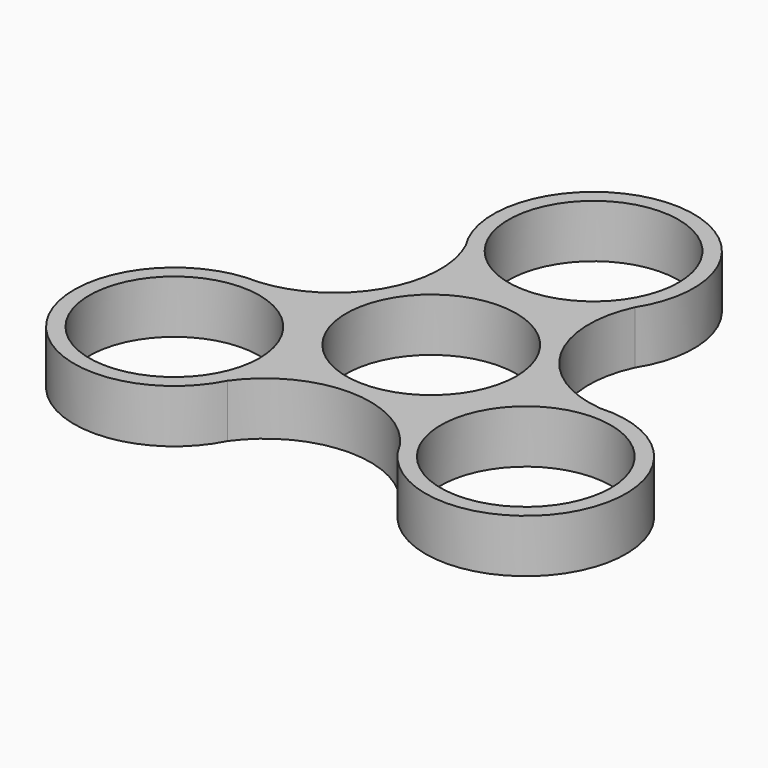
from build123d import *

# Parameters (mm, degrees)
F0_R     = 11.2
F1_DEPTH = 7
F2_R     = 1.5
F3_DEPTH = 7


# Not quite as in the source:
# - a feature names something its author has since deleted; it is built from what else it names


with BuildPart() as f1:
    # F0 (on Top) → F1 (new body)
    with BuildSketch(Plane.XY):
        with BuildLine():
            ThreePointArc((22.3972222345, -0.1780444605), (11.6219084102, 6.8053952105), (11.1419447663, 19.6368196267))
            ThreePointArc((11.1419447663, 19.6368196267), (-0.0899760733, 39.914441113), (-11.0444200915, 19.4855856595))
            ThreePointArc((-11.0444200915, 19.4855856595), (-11.7045993402, 6.6621703185), (-22.5769570295, -0.1692025982))
            ThreePointArc((-22.5769570295, -0.1692025982), (-34.5219319451, -20.0351421217), (-11.352802143, -19.3075411991))
            ThreePointArc((-11.352802143, -19.3075411991), (0.08269093, -13.467565529), (11.4350122631, -19.4676170286))
            ThreePointArc((11.4350122631, -19.4676170286), (34.6119080183, -19.8792989913), (22.3972222345, -0.1780444605))
        make_face()
        with Locations((-23.1356502259, -13.3573738858)):
            Circle(F0_R, mode=Mode.SUBTRACT)
        with Locations((23.1356502259, -13.3573738858)):
            Circle(F0_R, mode=Mode.SUBTRACT)
        Circle(F0_R, mode=Mode.SUBTRACT)
        with Locations((0, 26.7147477716)):
            Circle(F0_R, mode=Mode.SUBTRACT)
    extrude(amount=F1_DEPTH)

    # F2 (call 1 of 2: OpenCascade refuses the feature's edges together)
    f2_edges = [f1.edges().sort_by_distance(p)[0] for p in [
        (-34.521932, -20.035142, 7),
        (-11.704599, 6.66217, 7),
        (34.611908, -19.879299, 7),
        (-0.089976, 39.914441, 7),
        (0.082691, -13.467566, 7),
        (11.621908, 6.805395, 7),
    ]]
    fillet(f2_edges, radius=F2_R)

    # F2#2 (call 2 of 2)
    f2_2_edges = [f1.edges().sort_by_distance(p)[0] for p in [
        (34.611908, -19.879299, 0),
        (0.082691, -13.467566, 0),
        (-34.521932, -20.035142, 0),
        (-0.089976, 39.914441, 0),
        (11.621908, 6.805395, 0),
        (-11.704599, 6.66217, 0),
    ]]
    fillet(f2_2_edges, radius=F2_R)

    # F0 (on Top) → F3 (join)
    with BuildSketch(Plane.XY):
        with BuildLine():
            ThreePointArc((22.3972222345, -0.1780444605), (11.6219084102, 6.8053952105), (11.1419447663, 19.6368196267))
            ThreePointArc((11.1419447663, 19.6368196267), (-0.0899760733, 39.914441113), (-11.0444200915, 19.4855856595))
            ThreePointArc((-11.0444200915, 19.4855856595), (-11.7045993402, 6.6621703185), (-22.5769570295, -0.1692025982))
            ThreePointArc((-22.5769570295, -0.1692025982), (-34.5219319451, -20.0351421217), (-11.352802143, -19.3075411991))
            ThreePointArc((-11.352802143, -19.3075411991), (0.08269093, -13.467565529), (11.4350122631, -19.4676170286))
            ThreePointArc((11.4350122631, -19.4676170286), (34.6119080183, -19.8792989913), (22.3972222345, -0.1780444605))
        make_face()
        with Locations((-23.1356502259, -13.3573738858)):
            Circle(F0_R, mode=Mode.SUBTRACT)
        with Locations((23.1356502259, -13.3573738858)):
            Circle(F0_R, mode=Mode.SUBTRACT)
        Circle(F0_R, mode=Mode.SUBTRACT)
        with Locations((0, 26.7147477716)):
            Circle(F0_R, mode=Mode.SUBTRACT)
    extrude(amount=F3_DEPTH)


solid = f1.part
